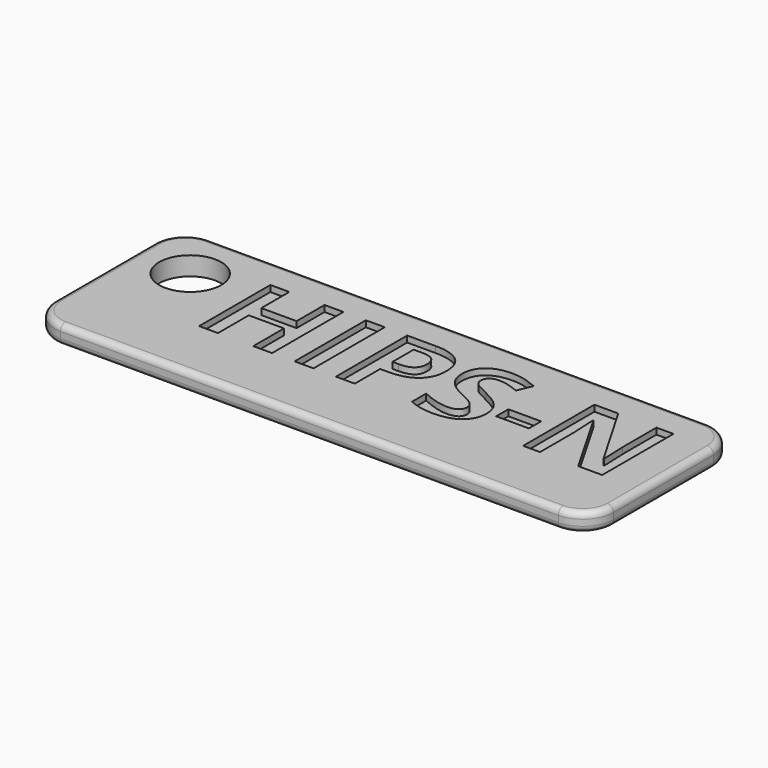
from build123d import *

# Parameters (mm, degrees)
F0_W         = 90
F0_H         = 30
F1_DEPTH     = 3
F2_R         = 1
F3_T1_DEPTH  = 3
F3_T4_ANGLE  = 90
F3_T6_ANGLE  = 90
F3_T8_ANGLE  = 90
F3_T10_ANGLE = 90
F3_T12_ANGLE = 90
F3_T14_ANGLE = 90
F3_T16_ANGLE = 90
F3_T18_ANGLE = 90
F4_R         = 5
F5_DEPTH     = 3
F6_TEXT_SIZE = 20.0904810267
F7_DEPTH     = 1


# Not quite as in the source:
# - a fillet or chamfer that OpenCascade refuses, or shapes differently, is made with other operations: its cross-section is extruded or revolved along the edge and cut away or added
# - Text() gives the source's letters only with a copy of the font that has no kerning and outlines rounded to 1/6400 em; it was checked with that copy


with BuildPart() as f1:
    # F0 (on Top) → F1 (new body)
    with BuildSketch(Plane.XY):
        Rectangle(F0_W, F0_H)
    extrude(amount=F1_DEPTH)

    # F2
    f2_edges = [f1.edges().sort_by_distance(p)[0] for p in [
        (0, 15, 3),
        (-45, 0, 3),
        (0, -15, 3),
        (45, 0, 3),
        (0, 15, 0),
        (-45, 0, 0),
        (0, -15, 0),
        (45, 0, 0),
    ]]
    fillet(f2_edges, radius=F2_R)

    # F3: fillet of radius 5 on 4 edges, made by hand

    # F3_s2 → F3_t1 (cut)
    with BuildSketch(Plane.XY):
        with BuildLine():
            ThreePointArc((45.0004, -9.9990343146), (43.5355339059, -13.5355339059), (39.9990343146, -15.0004))
            Line((39.9990343146, -15.0004), (39.9990343146, -15.5005365685))
            ThreePointArc((39.9990343146, -15.5005365685), (42.4995171573, -15.5001365685), (45, -15.5001365685))
            Line((45, -15.5001365685), (45.5001365685, -15))
            ThreePointArc((45.5001365685, -15), (45.5001365685, -12.4995171573), (45.5005365685, -9.9990343146))
            Line((45.5005365685, -9.9990343146), (45.0004, -9.9990343146))
        make_face()
        with BuildLine():
            ThreePointArc((39.9990343146, 15.0004), (43.5355339059, 13.5355339059), (45.0004, 9.9990343146))
            Line((45.0004, 9.9990343146), (45.5005365685, 9.9990343146))
            ThreePointArc((45.5005365685, 9.9990343146), (45.5001365685, 12.4995171573), (45.5001365685, 15))
            Line((45.5001365685, 15), (45, 15.5001365685))
            ThreePointArc((45, 15.5001365685), (42.4995171573, 15.5001365685), (39.9990343146, 15.5005365685))
            Line((39.9990343146, 15.5005365685), (39.9990343146, 15.0004))
        make_face()
        with BuildLine():
            ThreePointArc((-39.9990343146, 15.0004), (-43.5355339059, 13.5355339059), (-45.0004, 9.9990343146))
            Line((-45.0004, 9.9990343146), (-45.5005365685, 9.9990343146))
            ThreePointArc((-45.5005365685, 9.9990343146), (-45.5001365685, 12.4995171573), (-45.5001365685, 15))
            Line((-45.5001365685, 15), (-45, 15.5001365685))
            ThreePointArc((-45, 15.5001365685), (-42.4995171573, 15.5001365685), (-39.9990343146, 15.5005365685))
            Line((-39.9990343146, 15.5005365685), (-39.9990343146, 15.0004))
        make_face()
        with BuildLine():
            ThreePointArc((-45.0004, -9.9990343146), (-43.5355339059, -13.5355339059), (-39.9990343146, -15.0004))
            Line((-39.9990343146, -15.0004), (-39.9990343146, -15.5005365685))
            ThreePointArc((-39.9990343146, -15.5005365685), (-42.4995171573, -15.5001365685), (-45, -15.5001365685))
            Line((-45, -15.5001365685), (-45.5001365685, -15))
            ThreePointArc((-45.5001365685, -15), (-45.5001365685, -12.4995171573), (-45.5005365685, -9.9990343146))
            Line((-45.5005365685, -9.9990343146), (-45.0004, -9.9990343146))
        make_face()
    extrude(amount=F3_T1_DEPTH, mode=Mode.SUBTRACT)

    # F3_s3 → F3_t4 (revolve, cut)
    with BuildSketch(Plane.YZ.offset(-39.9990343146)):
        with BuildLine():
            ThreePointArc((-14.0004, 0), (-14.7075067812, 0.2928932188), (-15.0004, 1))
            Line((-15.0004, 1), (-15.0004, 0))
            Line((-15.0004, 0), (-14.0004, 0))
        make_face()
    revolve(axis=Axis((-39.9990343146, -9.9990343146, 0), (0, 0, -1)), revolution_arc=F3_T4_ANGLE, mode=Mode.SUBTRACT)

    # F3_s5 → F3_t6 (revolve, cut)
    with BuildSketch(Plane.XZ.offset(9.9990343146)):
        with BuildLine():
            ThreePointArc((-44.0004, 3), (-44.7075067812, 2.7071067812), (-45.0004, 2))
            Line((-45.0004, 2), (-45.0004, 3))
            Line((-45.0004, 3), (-44.0004, 3))
        make_face()
    revolve(axis=Axis((-39.9990343146, -9.9990343146, 3), (0, 0, 1)), revolution_arc=F3_T6_ANGLE, mode=Mode.SUBTRACT)

    # F3_s7 → F3_t8 (revolve, cut)
    with BuildSketch(Plane.XZ.offset(-9.9990343146)):
        with BuildLine():
            ThreePointArc((-44.0004, 0), (-44.7075067812, 0.2928932188), (-45.0004, 1))
            Line((-45.0004, 1), (-45.0004, 0))
            Line((-45.0004, 0), (-44.0004, 0))
        make_face()
    revolve(axis=Axis((-39.9990343146, 9.9990343146, 0), (0, 0, -1)), revolution_arc=F3_T8_ANGLE, mode=Mode.SUBTRACT)

    # F3_s9 → F3_t10 (revolve, cut)
    with BuildSketch(Plane.YZ.offset(-39.9990343146)):
        with BuildLine():
            ThreePointArc((14.0004, 3), (14.7075067812, 2.7071067812), (15.0004, 2))
            Line((15.0004, 2), (15.0004, 3))
            Line((15.0004, 3), (14.0004, 3))
        make_face()
    revolve(axis=Axis((-39.9990343146, 9.9990343146, 3), (0, 0, 1)), revolution_arc=F3_T10_ANGLE, mode=Mode.SUBTRACT)

    # F3_s11 → F3_t12 (revolve, cut)
    with BuildSketch(Plane.YZ.offset(39.9990343146)):
        with BuildLine():
            ThreePointArc((14.0004, 0), (14.7075067812, 0.2928932188), (15.0004, 1))
            Line((15.0004, 1), (15.0004, 0))
            Line((15.0004, 0), (14.0004, 0))
        make_face()
    revolve(axis=Axis((39.9990343146, 9.9990343146, 0), (0, 0, -1)), revolution_arc=F3_T12_ANGLE, mode=Mode.SUBTRACT)

    # F3_s13 → F3_t14 (revolve, cut)
    with BuildSketch(Plane.XZ.offset(-9.9990343146)):
        with BuildLine():
            ThreePointArc((44.0004, 3), (44.7075067812, 2.7071067812), (45.0004, 2))
            Line((45.0004, 2), (45.0004, 3))
            Line((45.0004, 3), (44.0004, 3))
        make_face()
    revolve(axis=Axis((39.9990343146, 9.9990343146, 3), (0, 0, 1)), revolution_arc=F3_T14_ANGLE, mode=Mode.SUBTRACT)

    # F3_s15 → F3_t16 (revolve, cut)
    with BuildSketch(Plane.XZ.offset(9.9990343146)):
        with BuildLine():
            ThreePointArc((44.0004, 0), (44.7075067812, 0.2928932188), (45.0004, 1))
            Line((45.0004, 1), (45.0004, 0))
            Line((45.0004, 0), (44.0004, 0))
        make_face()
    revolve(axis=Axis((39.9990343146, -9.9990343146, 0), (0, 0, -1)), revolution_arc=F3_T16_ANGLE, mode=Mode.SUBTRACT)

    # F3_s17 → F3_t18 (revolve, cut)
    with BuildSketch(Plane.YZ.offset(39.9990343146)):
        with BuildLine():
            ThreePointArc((-14.0004, 3), (-14.7075067812, 2.7071067812), (-15.0004, 2))
            Line((-15.0004, 2), (-15.0004, 3))
            Line((-15.0004, 3), (-14.0004, 3))
        make_face()
    revolve(axis=Axis((39.9990343146, -9.9990343146, 3), (0, 0, 1)), revolution_arc=F3_T18_ANGLE, mode=Mode.SUBTRACT)

    # F4 (on face) → F5 (cut)
    with BuildSketch(Plane.XY.offset(3)):
        with Locations((-36, 6)):
            Circle(F4_R)
    extrude(amount=-F5_DEPTH, mode=Mode.SUBTRACT)

    # F6 (on face) → F7 (cut)
    with BuildSketch(Plane.XY.offset(3)):
        with Locations((-28, -4.4651463392)):
            Text('HIPS-N', F6_TEXT_SIZE, font='Open Sans', font_style=FontStyle.BOLD, text_align=(TextAlign.LEFT, TextAlign.BOTTOM))
    extrude(amount=-F7_DEPTH, mode=Mode.SUBTRACT)


solid = f1.part
